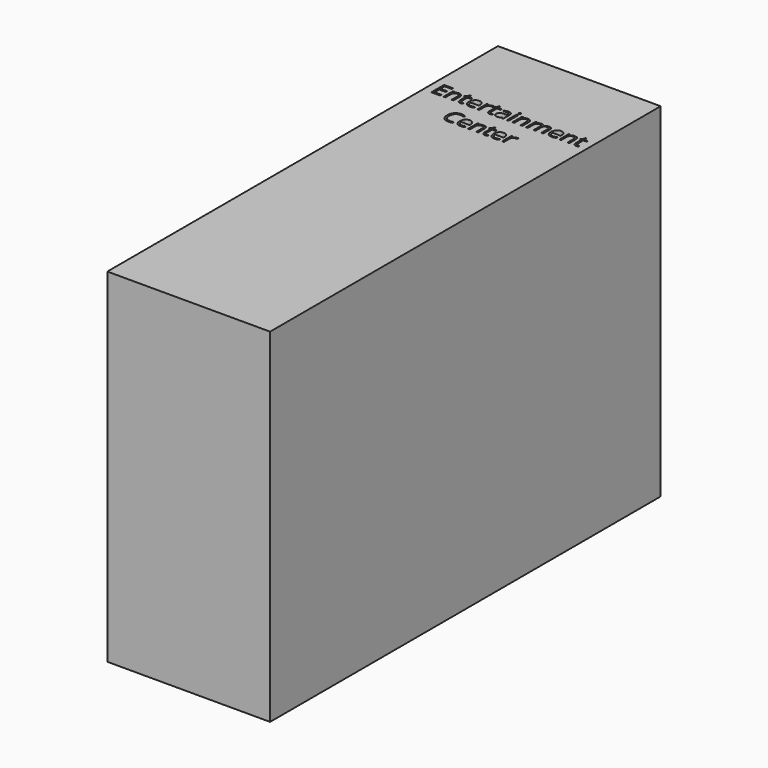
from build123d import *

# Parameters (mm, degrees)
F0_W     = 685.8
F0_H     = 2057.4
F0_W_2   = 7.6064578669
F0_H_2   = 50.1967595264
F1_DEPTH = 1447.8


with BuildPart() as f1:
    # F0 (on Top) → F1 (new body)
    with BuildSketch(Plane.XY):
        Rectangle(F0_W, F0_H)
        Polygon((-270.9672375193, 641.7474361589), (-270.9672375193, 634.785841772), (-308.2960394211, 634.785841772), (-308.2960394211, 701.7490517796), (-270.9672375193, 701.7490517796), (-270.9672375193, 694.8314253573), (-300.513709696, 694.8314253573), (-300.513709696, 673.2578107521), (-272.7552680776, 673.2578107521), (-272.7552680776, 666.3841522943), (-300.513709696, 666.3841522943), (-300.513709696, 641.7474361589), align=None, mode=Mode.SUBTRACT)
        with BuildLine():
            Line((-215.3184503889, 634.785841772), (-222.9249082558, 634.785841772))
            Line((-222.9249082558, 634.785841772), (-222.9249082558, 667.2635115853))
            add(Edge.make_bspline(
                [(-222.9249082558, 667.2635115853), (-222.9249082558, 673.3897146457), (-225.7168740047, 676.4161762055)],
                knots=[0, 0, 0, 1, 1, 1], degree=2))
            add(Edge.make_bspline(
                [(-225.7168740047, 676.4161762055), (-228.5088397535, 679.4426377653), (-234.4738269439, 679.4426377653)],
                knots=[0, 0, 0, 1, 1, 1], degree=2))
            add(Edge.make_bspline(
                [(-234.4738269439, 679.4426377653), (-242.3440925981, 679.4426377653), (-246.0080896439, 675.1850731981)],
                knots=[0, 0, 0, 1, 1, 1], degree=2))
            add(Edge.make_bspline(
                [(-246.0080896439, 675.1850731981), (-249.6720866896, 670.927508631), (-249.6720866896, 661.1226525367)],
                knots=[0, 0, 0, 1, 1, 1], degree=2))
            Line((-249.6720866896, 661.1226525367), (-249.6720866896, 634.785841772))
            Line((-249.6720866896, 634.785841772), (-257.2785445565, 634.785841772))
            Line((-257.2785445565, 634.785841772), (-257.2785445565, 684.9826012984))
            Line((-257.2785445565, 684.9826012984), (-251.0937175433, 684.9826012984))
            Line((-251.0937175433, 684.9826012984), (-249.862614536, 678.1089428406))
            Line((-249.862614536, 678.1089428406), (-249.4962148314, 678.1089428406))
            add(Edge.make_bspline(
                [(-249.4962148314, 678.1089428406), (-247.1512567221, 681.8169078509), (-242.9376601196, 683.8614182024)],
                knots=[0, 0, 0, 1, 1, 1], degree=2))
            add(Edge.make_bspline(
                [(-242.9376601196, 683.8614182024), (-238.724063517, 685.9059285539), (-233.5504996884, 685.9059285539)],
                knots=[0, 0, 0, 1, 1, 1], degree=2))
            add(Edge.make_bspline(
                [(-233.5504996884, 685.9059285539), (-224.4784430032, 685.9059285539), (-219.8984466961, 681.5311160813)],
                knots=[0, 0, 0, 1, 1, 1], degree=2))
            add(Edge.make_bspline(
                [(-219.8984466961, 681.5311160813), (-215.3184503889, 677.1563036087), (-215.3184503889, 667.5273193726)],
                knots=[0, 0, 0, 1, 1, 1], degree=2))
            Line((-215.3184503889, 667.5273193726), (-215.3184503889, 634.785841772))
        make_face(mode=Mode.SUBTRACT)
        with BuildLine():
            add(Edge.make_bspline(
                [(-189.4066632816, 642.5754994912), (-187.2522330187, 640.1499334469), (-183.5003000439, 640.1499334469)],
                knots=[0, 0, 0, 1, 1, 1], degree=2))
            add(Edge.make_bspline(
                [(-183.5003000439, 640.1499334469), (-181.4777736746, 640.1499334469), (-179.6018071872, 640.4430532106)],
                knots=[0, 0, 0, 1, 1, 1], degree=2))
            add(Edge.make_bspline(
                [(-179.6018071872, 640.4430532106), (-177.7258406998, 640.7361729743), (-176.6266415861, 641.0586047143)],
                knots=[0, 0, 0, 1, 1, 1], degree=2))
            Line((-176.6266415861, 641.0586047143), (-176.6266415861, 635.2401774057))
            add(Edge.make_bspline(
                [(-176.6266415861, 635.2401774057), (-177.8577445934, 634.6539378784), (-180.2613266554, 634.2582261974)],
                knots=[0, 0, 0, 1, 1, 1], degree=2))
            add(Edge.make_bspline(
                [(-180.2613266554, 634.2582261974), (-182.6649087174, 633.8625145165), (-184.5994991576, 633.8625145165)],
                knots=[0, 0, 0, 1, 1, 1], degree=2))
            add(Edge.make_bspline(
                [(-184.5994991576, 633.8625145165), (-199.1528954232, 633.8625145165), (-199.1528954232, 649.207334144)],
                knots=[0, 0, 0, 1, 1, 1], degree=2))
            Line((-199.1528954232, 649.207334144), (-199.1528954232, 679.0762380607))
            Line((-199.1528954232, 679.0762380607), (-206.348985621, 679.0762380607))
            Line((-206.348985621, 679.0762380607), (-206.348985621, 682.7402351064))
            Line((-206.348985621, 682.7402351064), (-199.1528954232, 685.9059285539))
            Line((-199.1528954232, 685.9059285539), (-195.9578899993, 696.6194559156))
            Line((-195.9578899993, 696.6194559156), (-191.5610935444, 696.6194559156))
            Line((-191.5610935444, 696.6194559156), (-191.5610935444, 684.9826012984))
            Line((-191.5610935444, 684.9826012984), (-176.9930412907, 684.9826012984))
            Line((-176.9930412907, 684.9826012984), (-176.9930412907, 679.0762380607))
            Line((-176.9930412907, 679.0762380607), (-191.5610935444, 679.0762380607))
            Line((-191.5610935444, 679.0762380607), (-191.5610935444, 649.529765884))
            add(Edge.make_bspline(
                [(-191.5610935444, 649.529765884), (-191.5610935444, 645.0010655355), (-189.4066632816, 642.5754994912)],
                knots=[0, 0, 0, 1, 1, 1], degree=2))
        make_face(mode=Mode.SUBTRACT)
        with BuildLine():
            add(Edge.make_bspline(
                [(-118.1785607127, 564.6129703523), (-125.7850185796, 568.1743754808), (-133.3914764466, 568.1743754808)],
                knots=[0, 0, 0, 1, 1, 1], degree=2))
            add(Edge.make_bspline(
                [(-133.3914764466, 568.1743754808), (-144.4274355483, 568.1743754808), (-150.817446396, 560.8243974071)],
                knots=[0, 0, 0, 1, 1, 1], degree=2))
            add(Edge.make_bspline(
                [(-150.817446396, 560.8243974071), (-157.2074572438, 553.4744193333), (-157.2074572438, 540.6943976379)],
                knots=[0, 0, 0, 1, 1, 1], degree=2))
            add(Edge.make_bspline(
                [(-157.2074572438, 540.6943976379), (-157.2074572438, 527.562632226), (-151.0446142128, 520.3885260105)],
                knots=[0, 0, 0, 1, 1, 1], degree=2))
            add(Edge.make_bspline(
                [(-151.0446142128, 520.3885260105), (-144.8817711819, 513.2144197949), (-133.4794123757, 513.2144197949)],
                knots=[0, 0, 0, 1, 1, 1], degree=2))
            add(Edge.make_bspline(
                [(-133.4794123757, 513.2144197949), (-126.4738500242, 513.2144197949), (-117.4897292681, 515.7352497624)],
                knots=[0, 0, 0, 1, 1, 1], degree=2))
            Line((-117.4897292681, 515.7352497624), (-117.4897292681, 508.9202152574))
            add(Edge.make_bspline(
                [(-117.4897292681, 508.9202152574), (-124.451323655, 506.2967933726), (-134.6665474185, 506.2967933726)],
                knots=[0, 0, 0, 1, 1, 1], degree=2))
            add(Edge.make_bspline(
                [(-134.6665474185, 506.2967933726), (-149.454439495, 506.2967933726), (-157.4932490133, 515.2809141287)],
                knots=[0, 0, 0, 1, 1, 1], degree=2))
            add(Edge.make_bspline(
                [(-157.4932490133, 515.2809141287), (-165.5320585316, 524.2650348848), (-165.5320585316, 540.7969895551)],
                knots=[0, 0, 0, 1, 1, 1], degree=2))
            add(Edge.make_bspline(
                [(-165.5320585316, 540.7969895551), (-165.5320585316, 551.1441172123), (-161.6628776513, 558.9264469374)],
                knots=[0, 0, 0, 1, 1, 1], degree=2))
            add(Edge.make_bspline(
                [(-161.6628776513, 558.9264469374), (-157.7936967711, 566.7087766625), (-150.4876866619, 570.9223732651)],
                knots=[0, 0, 0, 1, 1, 1], degree=2))
            add(Edge.make_bspline(
                [(-150.4876866619, 570.9223732651), (-143.1816765527, 575.1359698677), (-133.2888845293, 575.1359698677)],
                knots=[0, 0, 0, 1, 1, 1], degree=2))
            add(Edge.make_bspline(
                [(-133.2888845293, 575.1359698677), (-122.765885014, 575.1359698677), (-114.8809633716, 571.2961009637)],
                knots=[0, 0, 0, 1, 1, 1], degree=2))
            Line((-114.8809633716, 571.2961009637), (-118.1785607127, 564.6129703523))
        make_face(mode=Mode.SUBTRACT)
        with BuildLine():
            add(Edge.make_bspline(
                [(-136.7183857641, 634.624625902), (-140.3091028689, 633.8625145165), (-145.3947307683, 633.8625145165)],
                knots=[0, 0, 0, 1, 1, 1], degree=2))
            add(Edge.make_bspline(
                [(-145.3947307683, 633.8625145165), (-156.5186257992, 633.8625145165), (-162.9599326055, 640.6482370452)],
                knots=[0, 0, 0, 1, 1, 1], degree=2))
            add(Edge.make_bspline(
                [(-162.9599326055, 640.6482370452), (-169.4012394119, 647.4339595738), (-169.4012394119, 659.466525872)],
                knots=[0, 0, 0, 1, 1, 1], degree=2))
            add(Edge.make_bspline(
                [(-169.4012394119, 659.466525872), (-169.4012394119, 671.6163400756), (-163.4215962333, 678.7611343148)],
                knots=[0, 0, 0, 1, 1, 1], degree=2))
            add(Edge.make_bspline(
                [(-163.4215962333, 678.7611343148), (-157.4419530547, 685.9059285539), (-147.3586331849, 685.9059285539)],
                knots=[0, 0, 0, 1, 1, 1], degree=2))
            add(Edge.make_bspline(
                [(-147.3586331849, 685.9059285539), (-137.9348327833, 685.9059285539), (-132.4388372147, 679.6991175585)],
                knots=[0, 0, 0, 1, 1, 1], degree=2))
            add(Edge.make_bspline(
                [(-132.4388372147, 679.6991175585), (-126.9428416461, 673.492306563), (-126.9428416461, 663.3210507641)],
                knots=[0, 0, 0, 1, 1, 1], degree=2))
            Line((-126.9428416461, 663.3210507641), (-126.9428416461, 658.5138866401))
            Line((-126.9428416461, 658.5138866401), (-161.5163177695, 658.5138866401))
            add(Edge.make_bspline(
                [(-161.5163177695, 658.5138866401), (-161.2818219586, 649.6763257658), (-157.0462413737, 645.0963294587)],
                knots=[0, 0, 0, 1, 1, 1], degree=2))
            add(Edge.make_bspline(
                [(-157.0462413737, 645.0963294587), (-152.8106607889, 640.5163331515), (-145.1162669929, 640.5163331515)],
                knots=[0, 0, 0, 1, 1, 1], degree=2))
            add(Edge.make_bspline(
                [(-145.1162669929, 640.5163331515), (-137.0115055277, 640.5163331515), (-129.097271909, 643.9018664218)],
                knots=[0, 0, 0, 1, 1, 1], degree=2))
            Line((-129.097271909, 643.9018664218), (-129.097271909, 637.1161438931))
            add(Edge.make_bspline(
                [(-129.097271909, 637.1161438931), (-133.1276686593, 635.3867372875), (-136.7183857641, 634.624625902)],
                knots=[0, 0, 0, 1, 1, 1], degree=2))
        make_face(mode=Mode.SUBTRACT)
        with BuildLine():
            add(Edge.make_bspline(
                [(-99.7266715905, 683.2458666987), (-95.7842107693, 685.9059285539), (-91.0649825744, 685.9059285539)],
                knots=[0, 0, 0, 1, 1, 1], degree=2))
            add(Edge.make_bspline(
                [(-91.0649825744, 685.9059285539), (-87.7234172687, 685.9059285539), (-85.0706834076, 685.349001003)],
                knots=[0, 0, 0, 1, 1, 1], degree=2))
            Line((-85.0706834076, 685.349001003), (-86.1259145567, 678.299470687))
            add(Edge.make_bspline(
                [(-86.1259145567, 678.299470687), (-89.2329840515, 678.9883021316), (-91.6219101253, 678.9883021316)],
                knots=[0, 0, 0, 1, 1, 1], degree=2))
            add(Edge.make_bspline(
                [(-91.6219101253, 678.9883021316), (-97.7188012094, 678.9883021316), (-102.0423177234, 674.0419061199)],
                knots=[0, 0, 0, 1, 1, 1], degree=2))
            add(Edge.make_bspline(
                [(-102.0423177234, 674.0419061199), (-106.3658342373, 669.0955101081), (-106.3658342373, 661.7235480522)],
                knots=[0, 0, 0, 1, 1, 1], degree=2))
            Line((-106.3658342373, 661.7235480522), (-106.3658342373, 634.785841772))
            Line((-106.3658342373, 634.785841772), (-113.9722921042, 634.785841772))
            Line((-113.9722921042, 634.785841772), (-113.9722921042, 684.9826012984))
            Line((-113.9722921042, 684.9826012984), (-107.699529162, 684.9826012984))
            Line((-107.699529162, 684.9826012984), (-106.820169871, 675.6907047904))
            Line((-106.820169871, 675.6907047904), (-106.4537701664, 675.6907047904))
            add(Edge.make_bspline(
                [(-106.4537701664, 675.6907047904), (-103.6691324117, 680.5858048435), (-99.7266715905, 683.2458666987)],
                knots=[0, 0, 0, 1, 1, 1], degree=2))
        make_face(mode=Mode.SUBTRACT)
        with BuildLine():
            add(Edge.make_bspline(
                [(-74.1373162231, 507.0589047581), (-77.7280333279, 506.2967933726), (-82.8136612274, 506.2967933726)],
                knots=[0, 0, 0, 1, 1, 1], degree=2))
            add(Edge.make_bspline(
                [(-82.8136612274, 506.2967933726), (-93.9375562582, 506.2967933726), (-100.3788630646, 513.0825159013)],
                knots=[0, 0, 0, 1, 1, 1], degree=2))
            add(Edge.make_bspline(
                [(-100.3788630646, 513.0825159013), (-106.820169871, 519.86823843), (-106.820169871, 531.9008047281)],
                knots=[0, 0, 0, 1, 1, 1], degree=2))
            add(Edge.make_bspline(
                [(-106.820169871, 531.9008047281), (-106.820169871, 544.0506189317), (-100.8405266924, 551.1954131709)],
                knots=[0, 0, 0, 1, 1, 1], degree=2))
            add(Edge.make_bspline(
                [(-100.8405266924, 551.1954131709), (-94.8608835137, 558.3402074101), (-84.7775636439, 558.3402074101)],
                knots=[0, 0, 0, 1, 1, 1], degree=2))
            add(Edge.make_bspline(
                [(-84.7775636439, 558.3402074101), (-75.3537632423, 558.3402074101), (-69.8577676737, 552.1333964146)],
                knots=[0, 0, 0, 1, 1, 1], degree=2))
            add(Edge.make_bspline(
                [(-69.8577676737, 552.1333964146), (-64.3617721052, 545.9265854192), (-64.3617721052, 535.7553296202)],
                knots=[0, 0, 0, 1, 1, 1], degree=2))
            Line((-64.3617721052, 535.7553296202), (-64.3617721052, 530.9481654962))
            Line((-64.3617721052, 530.9481654962), (-98.9352482286, 530.9481654962))
            add(Edge.make_bspline(
                [(-98.9352482286, 530.9481654962), (-98.7007524177, 522.110604622), (-94.4651718328, 517.5306083148)],
                knots=[0, 0, 0, 1, 1, 1], degree=2))
            add(Edge.make_bspline(
                [(-94.4651718328, 517.5306083148), (-90.229591248, 512.9506120077), (-82.5351974519, 512.9506120077)],
                knots=[0, 0, 0, 1, 1, 1], degree=2))
            add(Edge.make_bspline(
                [(-82.5351974519, 512.9506120077), (-74.4304359868, 512.9506120077), (-66.516202368, 516.3361452779)],
                knots=[0, 0, 0, 1, 1, 1], degree=2))
            Line((-66.516202368, 516.3361452779), (-66.516202368, 509.5504227492))
            add(Edge.make_bspline(
                [(-66.516202368, 509.5504227492), (-70.5465991183, 507.8210161436), (-74.1373162231, 507.0589047581)],
                knots=[0, 0, 0, 1, 1, 1], degree=2))
        make_face(mode=Mode.SUBTRACT)
        with BuildLine():
            Line((-9.4311283957, 507.2201206281), (-17.0375862626, 507.2201206281))
            Line((-17.0375862626, 507.2201206281), (-17.0375862626, 539.6977904414))
            add(Edge.make_bspline(
                [(-17.0375862626, 539.6977904414), (-17.0375862626, 545.8239935019), (-19.8295520114, 548.8504550616)],
                knots=[0, 0, 0, 1, 1, 1], degree=2))
            add(Edge.make_bspline(
                [(-19.8295520114, 548.8504550616), (-22.6215177603, 551.8769166214), (-28.5865049507, 551.8769166214)],
                knots=[0, 0, 0, 1, 1, 1], degree=2))
            add(Edge.make_bspline(
                [(-28.5865049507, 551.8769166214), (-36.4567706049, 551.8769166214), (-40.1207676507, 547.6193520543)],
                knots=[0, 0, 0, 1, 1, 1], degree=2))
            add(Edge.make_bspline(
                [(-40.1207676507, 547.6193520543), (-43.7847646964, 543.3617874871), (-43.7847646964, 533.5569313928)],
                knots=[0, 0, 0, 1, 1, 1], degree=2))
            Line((-43.7847646964, 533.5569313928), (-43.7847646964, 507.2201206281))
            Line((-43.7847646964, 507.2201206281), (-51.3912225633, 507.2201206281))
            Line((-51.3912225633, 507.2201206281), (-51.3912225633, 557.4168801545))
            Line((-51.3912225633, 557.4168801545), (-45.2063955501, 557.4168801545))
            Line((-45.2063955501, 557.4168801545), (-43.9752925428, 550.5432216968))
            Line((-43.9752925428, 550.5432216968), (-43.6088928382, 550.5432216968))
            add(Edge.make_bspline(
                [(-43.6088928382, 550.5432216968), (-41.2639347289, 554.251186707), (-37.0503381263, 556.2956970585)],
                knots=[0, 0, 0, 1, 1, 1], degree=2))
            add(Edge.make_bspline(
                [(-37.0503381263, 556.2956970585), (-32.8367415238, 558.3402074101), (-27.6631776952, 558.3402074101)],
                knots=[0, 0, 0, 1, 1, 1], degree=2))
            add(Edge.make_bspline(
                [(-27.6631776952, 558.3402074101), (-18.59112101, 558.3402074101), (-14.0111247028, 553.9653949375)],
                knots=[0, 0, 0, 1, 1, 1], degree=2))
            add(Edge.make_bspline(
                [(-14.0111247028, 553.9653949375), (-9.4311283957, 549.5905824649), (-9.4311283957, 539.9615982287)],
                knots=[0, 0, 0, 1, 1, 1], degree=2))
            Line((-9.4311283957, 539.9615982287), (-9.4311283957, 507.2201206281))
        make_face(mode=Mode.SUBTRACT)
        with BuildLine():
            add(Edge.make_bspline(
                [(-65.3730352898, 642.5754994912), (-63.2186050269, 640.1499334469), (-59.4666720521, 640.1499334469)],
                knots=[0, 0, 0, 1, 1, 1], degree=2))
            add(Edge.make_bspline(
                [(-59.4666720521, 640.1499334469), (-57.4441456828, 640.1499334469), (-55.5681791954, 640.4430532106)],
                knots=[0, 0, 0, 1, 1, 1], degree=2))
            add(Edge.make_bspline(
                [(-55.5681791954, 640.4430532106), (-53.692212708, 640.7361729743), (-52.5930135943, 641.0586047143)],
                knots=[0, 0, 0, 1, 1, 1], degree=2))
            Line((-52.5930135943, 641.0586047143), (-52.5930135943, 635.2401774057))
            add(Edge.make_bspline(
                [(-52.5930135943, 635.2401774057), (-53.8241166017, 634.6539378784), (-56.2276986637, 634.2582261974)],
                knots=[0, 0, 0, 1, 1, 1], degree=2))
            add(Edge.make_bspline(
                [(-56.2276986637, 634.2582261974), (-58.6312807256, 633.8625145165), (-60.5658711658, 633.8625145165)],
                knots=[0, 0, 0, 1, 1, 1], degree=2))
            add(Edge.make_bspline(
                [(-60.5658711658, 633.8625145165), (-75.1192674314, 633.8625145165), (-75.1192674314, 649.207334144)],
                knots=[0, 0, 0, 1, 1, 1], degree=2))
            Line((-75.1192674314, 649.207334144), (-75.1192674314, 679.0762380607))
            Line((-75.1192674314, 679.0762380607), (-82.3153576292, 679.0762380607))
            Line((-82.3153576292, 679.0762380607), (-82.3153576292, 682.7402351064))
            Line((-82.3153576292, 682.7402351064), (-75.1192674314, 685.9059285539))
            Line((-75.1192674314, 685.9059285539), (-71.9242620075, 696.6194559156))
            Line((-71.9242620075, 696.6194559156), (-67.5274655527, 696.6194559156))
            Line((-67.5274655527, 696.6194559156), (-67.5274655527, 684.9826012984))
            Line((-67.5274655527, 684.9826012984), (-52.9594132989, 684.9826012984))
            Line((-52.9594132989, 684.9826012984), (-52.9594132989, 679.0762380607))
            Line((-52.9594132989, 679.0762380607), (-67.5274655527, 679.0762380607))
            Line((-67.5274655527, 679.0762380607), (-67.5274655527, 649.529765884))
            add(Edge.make_bspline(
                [(-67.5274655527, 649.529765884), (-67.5274655527, 645.0010655355), (-65.3730352898, 642.5754994912)],
                knots=[0, 0, 0, 1, 1, 1], degree=2))
        make_face(mode=Mode.SUBTRACT)
        with BuildLine():
            Line((-6.0602511136, 634.785841772), (-11.702806564, 634.785841772))
            Line((-11.702806564, 634.785841772), (-13.2123733469, 641.9379640053))
            Line((-13.2123733469, 641.9379640053), (-13.5787730514, 641.9379640053))
            add(Edge.make_bspline(
                [(-13.5787730514, 641.9379640053), (-17.3307060263, 637.2187358104), (-21.0606550188, 635.5406251634)],
                knots=[0, 0, 0, 1, 1, 1], degree=2))
            add(Edge.make_bspline(
                [(-21.0606550188, 635.5406251634), (-24.7906040114, 633.8625145165), (-30.3891914972, 633.8625145165)],
                knots=[0, 0, 0, 1, 1, 1], degree=2))
            add(Edge.make_bspline(
                [(-30.3891914972, 633.8625145165), (-37.8490894823, 633.8625145165), (-42.0846700672, 637.7170394086)],
                knots=[0, 0, 0, 1, 1, 1], degree=2))
            add(Edge.make_bspline(
                [(-42.0846700672, 637.7170394086), (-46.320250652, 641.5715643007), (-46.320250652, 648.6650625812)],
                knots=[0, 0, 0, 1, 1, 1], degree=2))
            add(Edge.make_bspline(
                [(-46.320250652, 648.6650625812), (-46.320250652, 663.8633223269), (-22.0059662566, 664.596121736)],
                knots=[0, 0, 0, 1, 1, 1], degree=2))
            Line((-22.0059662566, 664.596121736), (-13.4908371223, 664.8745855115))
            Line((-13.4908371223, 664.8745855115), (-13.4908371223, 667.9963109944))
            add(Edge.make_bspline(
                [(-13.4908371223, 667.9963109944), (-13.4908371223, 673.9026742321), (-16.026323078, 676.7166239633)],
                knots=[0, 0, 0, 1, 1, 1], degree=2))
            add(Edge.make_bspline(
                [(-16.026323078, 676.7166239633), (-18.5618090336, 679.5305736944), (-24.1603965195, 679.5305736944)],
                knots=[0, 0, 0, 1, 1, 1], degree=2))
            add(Edge.make_bspline(
                [(-24.1603965195, 679.5305736944), (-30.4331594618, 679.5305736944), (-38.3473930805, 675.6907047904)],
                knots=[0, 0, 0, 1, 1, 1], degree=2))
            Line((-38.3473930805, 675.6907047904), (-40.6923511898, 681.5091320991))
            add(Edge.make_bspline(
                [(-40.6923511898, 681.5091320991), (-36.9843861795, 683.5170024801), (-32.5656057424, 684.6601695584)],
                knots=[0, 0, 0, 1, 1, 1], degree=2))
            add(Edge.make_bspline(
                [(-32.5656057424, 684.6601695584), (-28.1468253052, 685.8033366366), (-23.6914048976, 685.8033366366)],
                knots=[0, 0, 0, 1, 1, 1], degree=2))
            add(Edge.make_bspline(
                [(-23.6914048976, 685.8033366366), (-14.7219401297, 685.8033366366), (-10.3910956217, 681.824235845)],
                knots=[0, 0, 0, 1, 1, 1], degree=2))
            add(Edge.make_bspline(
                [(-10.3910956217, 681.824235845), (-6.0602511136, 677.8451350533), (-6.0602511136, 669.0515421436)],
                knots=[0, 0, 0, 1, 1, 1], degree=2))
            Line((-6.0602511136, 669.0515421436), (-6.0602511136, 634.785841772))
        make_face(mode=Mode.SUBTRACT)
        with BuildLine():
            add(Edge.make_bspline(
                [(16.4806587117, 515.0097783474), (18.6350889745, 512.5842123031), (22.3870219494, 512.5842123031)],
                knots=[0, 0, 0, 1, 1, 1], degree=2))
            add(Edge.make_bspline(
                [(22.3870219494, 512.5842123031), (24.4095483186, 512.5842123031), (26.285514806, 512.8773320667)],
                knots=[0, 0, 0, 1, 1, 1], degree=2))
            add(Edge.make_bspline(
                [(26.285514806, 512.8773320667), (28.1614812934, 513.1704518304), (29.2606804071, 513.4928835704)],
                knots=[0, 0, 0, 1, 1, 1], degree=2))
            Line((29.2606804071, 513.4928835704), (29.2606804071, 507.6744562618))
            add(Edge.make_bspline(
                [(29.2606804071, 507.6744562618), (28.0295773998, 507.0882167345), (25.6259953378, 506.6925050536)],
                knots=[0, 0, 0, 1, 1, 1], degree=2))
            add(Edge.make_bspline(
                [(25.6259953378, 506.6925050536), (23.2224132758, 506.2967933726), (21.2878228356, 506.2967933726)],
                knots=[0, 0, 0, 1, 1, 1], degree=2))
            add(Edge.make_bspline(
                [(21.2878228356, 506.2967933726), (6.73442657, 506.2967933726), (6.73442657, 521.6416130001)],
                knots=[0, 0, 0, 1, 1, 1], degree=2))
            Line((6.73442657, 521.6416130001), (6.73442657, 551.5105169168))
            Line((6.73442657, 551.5105169168), (-0.4616636278, 551.5105169168))
            Line((-0.4616636278, 551.5105169168), (-0.4616636278, 555.1745139626))
            Line((-0.4616636278, 555.1745139626), (6.73442657, 558.3402074101))
            Line((6.73442657, 558.3402074101), (9.9294319939, 569.0537347718))
            Line((9.9294319939, 569.0537347718), (14.3262284488, 569.0537347718))
            Line((14.3262284488, 569.0537347718), (14.3262284488, 557.4168801545))
            Line((14.3262284488, 557.4168801545), (28.8942807026, 557.4168801545))
            Line((28.8942807026, 557.4168801545), (28.8942807026, 551.5105169168))
            Line((28.8942807026, 551.5105169168), (14.3262284488, 551.5105169168))
            Line((14.3262284488, 551.5105169168), (14.3262284488, 521.9640447401))
            add(Edge.make_bspline(
                [(14.3262284488, 521.9640447401), (14.3262284488, 517.4353443916), (16.4806587117, 515.0097783474)],
                knots=[0, 0, 0, 1, 1, 1], degree=2))
        make_face(mode=Mode.SUBTRACT)
        with BuildLine():
            add(Edge.make_bspline(
                [(69.1689362291, 507.0589047581), (65.5782191243, 506.2967933726), (60.4925912249, 506.2967933726)],
                knots=[0, 0, 0, 1, 1, 1], degree=2))
            add(Edge.make_bspline(
                [(60.4925912249, 506.2967933726), (49.3686961941, 506.2967933726), (42.9273893877, 513.0825159013)],
                knots=[0, 0, 0, 1, 1, 1], degree=2))
            add(Edge.make_bspline(
                [(42.9273893877, 513.0825159013), (36.4860825813, 519.86823843), (36.4860825813, 531.9008047281)],
                knots=[0, 0, 0, 1, 1, 1], degree=2))
            add(Edge.make_bspline(
                [(36.4860825813, 531.9008047281), (36.4860825813, 544.0506189317), (42.4657257599, 551.1954131709)],
                knots=[0, 0, 0, 1, 1, 1], degree=2))
            add(Edge.make_bspline(
                [(42.4657257599, 551.1954131709), (48.4453689385, 558.3402074101), (58.5286888084, 558.3402074101)],
                knots=[0, 0, 0, 1, 1, 1], degree=2))
            add(Edge.make_bspline(
                [(58.5286888084, 558.3402074101), (67.95248921, 558.3402074101), (73.4484847785, 552.1333964146)],
                knots=[0, 0, 0, 1, 1, 1], degree=2))
            add(Edge.make_bspline(
                [(73.4484847785, 552.1333964146), (78.9444803471, 545.9265854192), (78.9444803471, 535.7553296202)],
                knots=[0, 0, 0, 1, 1, 1], degree=2))
            Line((78.9444803471, 535.7553296202), (78.9444803471, 530.9481654962))
            Line((78.9444803471, 530.9481654962), (44.3710042237, 530.9481654962))
            add(Edge.make_bspline(
                [(44.3710042237, 530.9481654962), (44.6055000346, 522.110604622), (48.8410806195, 517.5306083148)],
                knots=[0, 0, 0, 1, 1, 1], degree=2))
            add(Edge.make_bspline(
                [(48.8410806195, 517.5306083148), (53.0766612043, 512.9506120077), (60.7710550003, 512.9506120077)],
                knots=[0, 0, 0, 1, 1, 1], degree=2))
            add(Edge.make_bspline(
                [(60.7710550003, 512.9506120077), (68.8758164655, 512.9506120077), (76.7900500842, 516.3361452779)],
                knots=[0, 0, 0, 1, 1, 1], degree=2))
            Line((76.7900500842, 516.3361452779), (76.7900500842, 509.5504227492))
            add(Edge.make_bspline(
                [(76.7900500842, 509.5504227492), (72.7596533339, 507.8210161436), (69.1689362291, 507.0589047581)],
                knots=[0, 0, 0, 1, 1, 1], degree=2))
        make_face(mode=Mode.SUBTRACT)
        with Locations((13.3955731992, 659.8842215352)):
            Rectangle(F0_W_2, F0_H_2, mode=Mode.SUBTRACT)
        with BuildLine():
            add(Edge.make_bspline(
                [(10.2298797517, 694.7581454164), (8.9474807857, 696.0185604001), (8.9474807857, 698.5833583321)],
                knots=[0, 0, 0, 1, 1, 1], degree=2))
            add(Edge.make_bspline(
                [(8.9474807857, 698.5833583321), (8.9474807857, 701.1921242287), (10.2298797517, 702.4085712479)],
                knots=[0, 0, 0, 1, 1, 1], degree=2))
            add(Edge.make_bspline(
                [(10.2298797517, 702.4085712479), (11.5122787177, 703.625018267), (13.4468691578, 703.625018267)],
                knots=[0, 0, 0, 1, 1, 1], degree=2))
            add(Edge.make_bspline(
                [(13.4468691578, 703.625018267), (15.2788676807, 703.625018267), (16.6052346112, 702.3865872656)],
                knots=[0, 0, 0, 1, 1, 1], degree=2))
            add(Edge.make_bspline(
                [(16.6052346112, 702.3865872656), (17.9316015418, 701.1481562641), (17.9316015418, 698.5833583321)],
                knots=[0, 0, 0, 1, 1, 1], degree=2))
            add(Edge.make_bspline(
                [(17.9316015418, 698.5833583321), (17.9316015418, 696.0185604001), (16.6052346112, 694.7581454164)],
                knots=[0, 0, 0, 1, 1, 1], degree=2))
            add(Edge.make_bspline(
                [(16.6052346112, 694.7581454164), (15.2788676807, 693.4977304327), (13.4468691578, 693.4977304327)],
                knots=[0, 0, 0, 1, 1, 1], degree=2))
            add(Edge.make_bspline(
                [(13.4468691578, 693.4977304327), (11.5122787177, 693.4977304327), (10.2298797517, 694.7581454164)],
                knots=[0, 0, 0, 1, 1, 1], degree=2))
        make_face(mode=Mode.SUBTRACT)
        with BuildLine():
            Line((75.2804833014, 634.785841772), (67.6740254345, 634.785841772))
            Line((67.6740254345, 634.785841772), (67.6740254345, 667.2635115853))
            add(Edge.make_bspline(
                [(67.6740254345, 667.2635115853), (67.6740254345, 673.3897146457), (64.8820596856, 676.4161762055)],
                knots=[0, 0, 0, 1, 1, 1], degree=2))
            add(Edge.make_bspline(
                [(64.8820596856, 676.4161762055), (62.0900939368, 679.4426377653), (56.1251067464, 679.4426377653)],
                knots=[0, 0, 0, 1, 1, 1], degree=2))
            add(Edge.make_bspline(
                [(56.1251067464, 679.4426377653), (48.2548410922, 679.4426377653), (44.5908440464, 675.1850731981)],
                knots=[0, 0, 0, 1, 1, 1], degree=2))
            add(Edge.make_bspline(
                [(44.5908440464, 675.1850731981), (40.9268470007, 670.927508631), (40.9268470007, 661.1226525367)],
                knots=[0, 0, 0, 1, 1, 1], degree=2))
            Line((40.9268470007, 661.1226525367), (40.9268470007, 634.785841772))
            Line((40.9268470007, 634.785841772), (33.3203891338, 634.785841772))
            Line((33.3203891338, 634.785841772), (33.3203891338, 684.9826012984))
            Line((33.3203891338, 684.9826012984), (39.505216147, 684.9826012984))
            Line((39.505216147, 684.9826012984), (40.7363191543, 678.1089428406))
            Line((40.7363191543, 678.1089428406), (41.1027188589, 678.1089428406))
            add(Edge.make_bspline(
                [(41.1027188589, 678.1089428406), (43.4476769682, 681.8169078509), (47.6612735708, 683.8614182024)],
                knots=[0, 0, 0, 1, 1, 1], degree=2))
            add(Edge.make_bspline(
                [(47.6612735708, 683.8614182024), (51.8748701733, 685.9059285539), (57.0484340019, 685.9059285539)],
                knots=[0, 0, 0, 1, 1, 1], degree=2))
            add(Edge.make_bspline(
                [(57.0484340019, 685.9059285539), (66.1204906871, 685.9059285539), (70.7004869943, 681.5311160813)],
                knots=[0, 0, 0, 1, 1, 1], degree=2))
            add(Edge.make_bspline(
                [(70.7004869943, 681.5311160813), (75.2804833014, 677.1563036087), (75.2804833014, 667.5273193726)],
                knots=[0, 0, 0, 1, 1, 1], degree=2))
            Line((75.2804833014, 667.5273193726), (75.2804833014, 634.785841772))
        make_face(mode=Mode.SUBTRACT)
        with BuildLine():
            add(Edge.make_bspline(
                [(106.1606504028, 555.6801455549), (110.1031112239, 558.3402074101), (114.8223394188, 558.3402074101)],
                knots=[0, 0, 0, 1, 1, 1], degree=2))
            add(Edge.make_bspline(
                [(114.8223394188, 558.3402074101), (118.1639047245, 558.3402074101), (120.8166385856, 557.7832798591)],
                knots=[0, 0, 0, 1, 1, 1], degree=2))
            Line((120.8166385856, 557.7832798591), (119.7614074365, 550.7337495431))
            add(Edge.make_bspline(
                [(119.7614074365, 550.7337495431), (116.6543379417, 551.4225809877), (114.2654118679, 551.4225809877)],
                knots=[0, 0, 0, 1, 1, 1], degree=2))
            add(Edge.make_bspline(
                [(114.2654118679, 551.4225809877), (108.1685207838, 551.4225809877), (103.8450042699, 546.476184976)],
                knots=[0, 0, 0, 1, 1, 1], degree=2))
            add(Edge.make_bspline(
                [(103.8450042699, 546.476184976), (99.5214877559, 541.5297889643), (99.5214877559, 534.1578269083)],
                knots=[0, 0, 0, 1, 1, 1], degree=2))
            Line((99.5214877559, 534.1578269083), (99.5214877559, 507.2201206281))
            Line((99.5214877559, 507.2201206281), (91.915029889, 507.2201206281))
            Line((91.915029889, 507.2201206281), (91.915029889, 557.4168801545))
            Line((91.915029889, 557.4168801545), (98.1877928313, 557.4168801545))
            Line((98.1877928313, 557.4168801545), (99.0671521222, 548.1249836466))
            Line((99.0671521222, 548.1249836466), (99.4335518268, 548.1249836466))
            add(Edge.make_bspline(
                [(99.4335518268, 548.1249836466), (102.2181895816, 553.0200836997), (106.1606504028, 555.6801455549)],
                knots=[0, 0, 0, 1, 1, 1], degree=2))
        make_face(mode=Mode.SUBTRACT)
        with BuildLine():
            Line((162.4689570014, 634.785841772), (154.8771551227, 634.785841772))
            Line((154.8771551227, 634.785841772), (154.8771551227, 667.4393834435))
            add(Edge.make_bspline(
                [(154.8771551227, 667.4393834435), (154.8771551227, 673.4483385985), (152.3123571907, 676.4454881819)],
                knots=[0, 0, 0, 1, 1, 1], degree=2))
            add(Edge.make_bspline(
                [(152.3123571907, 676.4454881819), (149.7475592587, 679.4426377653), (144.3394996192, 679.4426377653)],
                knots=[0, 0, 0, 1, 1, 1], degree=2))
            add(Edge.make_bspline(
                [(144.3394996192, 679.4426377653), (137.2460013387, 679.4426377653), (133.8531400743, 675.3682730504)],
                knots=[0, 0, 0, 1, 1, 1], degree=2))
            add(Edge.make_bspline(
                [(133.8531400743, 675.3682730504), (130.46027881, 671.2939083356), (130.46027881, 662.8227471659)],
                knots=[0, 0, 0, 1, 1, 1], degree=2))
            Line((130.46027881, 662.8227471659), (130.46027881, 634.785841772))
            Line((130.46027881, 634.785841772), (122.8538209431, 634.785841772))
            Line((122.8538209431, 634.785841772), (122.8538209431, 667.4393834435))
            add(Edge.make_bspline(
                [(122.8538209431, 667.4393834435), (122.8538209431, 673.4483385985), (120.2890230111, 676.4454881819)],
                knots=[0, 0, 0, 1, 1, 1], degree=2))
            add(Edge.make_bspline(
                [(120.2890230111, 676.4454881819), (117.7242250791, 679.4426377653), (112.272197475, 679.4426377653)],
                knots=[0, 0, 0, 1, 1, 1], degree=2))
            add(Edge.make_bspline(
                [(112.272197475, 679.4426377653), (105.1347312299, 679.4426377653), (101.8151499065, 675.1630892159)],
                knots=[0, 0, 0, 1, 1, 1], degree=2))
            add(Edge.make_bspline(
                [(101.8151499065, 675.1630892159), (98.4955685831, 670.8835406665), (98.4955685831, 661.1226525367)],
                knots=[0, 0, 0, 1, 1, 1], degree=2))
            Line((98.4955685831, 661.1226525367), (98.4955685831, 634.785841772))
            Line((98.4955685831, 634.785841772), (90.8891107162, 634.785841772))
            Line((90.8891107162, 634.785841772), (90.8891107162, 684.9826012984))
            Line((90.8891107162, 684.9826012984), (97.0739377294, 684.9826012984))
            Line((97.0739377294, 684.9826012984), (98.3050407367, 678.1089428406))
            Line((98.3050407367, 678.1089428406), (98.6714404413, 678.1089428406))
            add(Edge.make_bspline(
                [(98.6714404413, 678.1089428406), (100.8258707042, 681.7729398863), (104.7463475431, 683.8394342201)],
                knots=[0, 0, 0, 1, 1, 1], degree=2))
            add(Edge.make_bspline(
                [(104.7463475431, 683.8394342201), (108.666824382, 685.9059285539), (113.5179564706, 685.9059285539)],
                knots=[0, 0, 0, 1, 1, 1], degree=2))
            add(Edge.make_bspline(
                [(113.5179564706, 685.9059285539), (125.2867149814, 685.9059285539), (128.9067440626, 677.3761434315)],
                knots=[0, 0, 0, 1, 1, 1], degree=2))
            Line((128.9067440626, 677.3761434315), (129.2731437672, 677.3761434315))
            add(Edge.make_bspline(
                [(129.2731437672, 677.3761434315), (131.5155099591, 681.3186042527), (135.7730745263, 683.6122664033)],
                knots=[0, 0, 0, 1, 1, 1], degree=2))
            add(Edge.make_bspline(
                [(135.7730745263, 683.6122664033), (140.0306390934, 685.9059285539), (145.4826666974, 685.9059285539)],
                knots=[0, 0, 0, 1, 1, 1], degree=2))
            add(Edge.make_bspline(
                [(145.4826666974, 685.9059285539), (153.9977958317, 685.9059285539), (158.2333764166, 681.5311160813)],
                knots=[0, 0, 0, 1, 1, 1], degree=2))
            add(Edge.make_bspline(
                [(158.2333764166, 681.5311160813), (162.4689570014, 677.1563036087), (162.4689570014, 667.5273193726)],
                knots=[0, 0, 0, 1, 1, 1], degree=2))
            Line((162.4689570014, 667.5273193726), (162.4689570014, 634.785841772))
        make_face(mode=Mode.SUBTRACT)
        with BuildLine():
            add(Edge.make_bspline(
                [(208.0197682738, 634.624625902), (204.429051169, 633.8625145165), (199.3434232696, 633.8625145165)],
                knots=[0, 0, 0, 1, 1, 1], degree=2))
            add(Edge.make_bspline(
                [(199.3434232696, 633.8625145165), (188.2195282387, 633.8625145165), (181.7782214324, 640.6482370452)],
                knots=[0, 0, 0, 1, 1, 1], degree=2))
            add(Edge.make_bspline(
                [(181.7782214324, 640.6482370452), (175.336914626, 647.4339595738), (175.336914626, 659.466525872)],
                knots=[0, 0, 0, 1, 1, 1], degree=2))
            add(Edge.make_bspline(
                [(175.336914626, 659.466525872), (175.336914626, 671.6163400756), (181.3165578046, 678.7611343148)],
                knots=[0, 0, 0, 1, 1, 1], degree=2))
            add(Edge.make_bspline(
                [(181.3165578046, 678.7611343148), (187.2962009832, 685.9059285539), (197.379520853, 685.9059285539)],
                knots=[0, 0, 0, 1, 1, 1], degree=2))
            add(Edge.make_bspline(
                [(197.379520853, 685.9059285539), (206.8033212546, 685.9059285539), (212.2993168232, 679.6991175585)],
                knots=[0, 0, 0, 1, 1, 1], degree=2))
            add(Edge.make_bspline(
                [(212.2993168232, 679.6991175585), (217.7953123918, 673.492306563), (217.7953123918, 663.3210507641)],
                knots=[0, 0, 0, 1, 1, 1], degree=2))
            Line((217.7953123918, 663.3210507641), (217.7953123918, 658.5138866401))
            Line((217.7953123918, 658.5138866401), (183.2218362684, 658.5138866401))
            add(Edge.make_bspline(
                [(183.2218362684, 658.5138866401), (183.4563320793, 649.6763257658), (187.6919126642, 645.0963294587)],
                knots=[0, 0, 0, 1, 1, 1], degree=2))
            add(Edge.make_bspline(
                [(187.6919126642, 645.0963294587), (191.927493249, 640.5163331515), (199.621887045, 640.5163331515)],
                knots=[0, 0, 0, 1, 1, 1], degree=2))
            add(Edge.make_bspline(
                [(199.621887045, 640.5163331515), (207.7266485102, 640.5163331515), (215.6408821289, 643.9018664218)],
                knots=[0, 0, 0, 1, 1, 1], degree=2))
            Line((215.6408821289, 643.9018664218), (215.6408821289, 637.1161438931))
            add(Edge.make_bspline(
                [(215.6408821289, 637.1161438931), (211.6104853786, 635.3867372875), (208.0197682738, 634.624625902)],
                knots=[0, 0, 0, 1, 1, 1], degree=2))
        make_face(mode=Mode.SUBTRACT)
        with BuildLine():
            Line((272.7259561013, 634.785841772), (265.1194982344, 634.785841772))
            Line((265.1194982344, 634.785841772), (265.1194982344, 667.2635115853))
            add(Edge.make_bspline(
                [(265.1194982344, 667.2635115853), (265.1194982344, 673.3897146457), (262.3275324855, 676.4161762055)],
                knots=[0, 0, 0, 1, 1, 1], degree=2))
            add(Edge.make_bspline(
                [(262.3275324855, 676.4161762055), (259.5355667367, 679.4426377653), (253.5705795462, 679.4426377653)],
                knots=[0, 0, 0, 1, 1, 1], degree=2))
            add(Edge.make_bspline(
                [(253.5705795462, 679.4426377653), (245.700313892, 679.4426377653), (242.0363168463, 675.1850731981)],
                knots=[0, 0, 0, 1, 1, 1], degree=2))
            add(Edge.make_bspline(
                [(242.0363168463, 675.1850731981), (238.3723198006, 670.927508631), (238.3723198006, 661.1226525367)],
                knots=[0, 0, 0, 1, 1, 1], degree=2))
            Line((238.3723198006, 661.1226525367), (238.3723198006, 634.785841772))
            Line((238.3723198006, 634.785841772), (230.7658619337, 634.785841772))
            Line((230.7658619337, 634.785841772), (230.7658619337, 684.9826012984))
            Line((230.7658619337, 684.9826012984), (236.9506889468, 684.9826012984))
            Line((236.9506889468, 684.9826012984), (238.1817919542, 678.1089428406))
            Line((238.1817919542, 678.1089428406), (238.5481916588, 678.1089428406))
            add(Edge.make_bspline(
                [(238.5481916588, 678.1089428406), (240.893149768, 681.8169078509), (245.1067463706, 683.8614182024)],
                knots=[0, 0, 0, 1, 1, 1], degree=2))
            add(Edge.make_bspline(
                [(245.1067463706, 683.8614182024), (249.3203429732, 685.9059285539), (254.4939068018, 685.9059285539)],
                knots=[0, 0, 0, 1, 1, 1], degree=2))
            add(Edge.make_bspline(
                [(254.4939068018, 685.9059285539), (263.565963487, 685.9059285539), (268.1459597941, 681.5311160813)],
                knots=[0, 0, 0, 1, 1, 1], degree=2))
            add(Edge.make_bspline(
                [(268.1459597941, 681.5311160813), (272.7259561013, 677.1563036087), (272.7259561013, 667.5273193726)],
                knots=[0, 0, 0, 1, 1, 1], degree=2))
            Line((272.7259561013, 667.5273193726), (272.7259561013, 634.785841772))
        make_face(mode=Mode.SUBTRACT)
        with BuildLine():
            add(Edge.make_bspline(
                [(298.6377432086, 642.5754994912), (300.7921734715, 640.1499334469), (304.5441064463, 640.1499334469)],
                knots=[0, 0, 0, 1, 1, 1], degree=2))
            add(Edge.make_bspline(
                [(304.5441064463, 640.1499334469), (306.5666328156, 640.1499334469), (308.442599303, 640.4430532106)],
                knots=[0, 0, 0, 1, 1, 1], degree=2))
            add(Edge.make_bspline(
                [(308.442599303, 640.4430532106), (310.3185657904, 640.7361729743), (311.4177649041, 641.0586047143)],
                knots=[0, 0, 0, 1, 1, 1], degree=2))
            Line((311.4177649041, 641.0586047143), (311.4177649041, 635.2401774057))
            add(Edge.make_bspline(
                [(311.4177649041, 635.2401774057), (310.1866618967, 634.6539378784), (307.7830798347, 634.2582261974)],
                knots=[0, 0, 0, 1, 1, 1], degree=2))
            add(Edge.make_bspline(
                [(307.7830798347, 634.2582261974), (305.3794977728, 633.8625145165), (303.4449073326, 633.8625145165)],
                knots=[0, 0, 0, 1, 1, 1], degree=2))
            add(Edge.make_bspline(
                [(303.4449073326, 633.8625145165), (288.891511067, 633.8625145165), (288.891511067, 649.207334144)],
                knots=[0, 0, 0, 1, 1, 1], degree=2))
            Line((288.891511067, 649.207334144), (288.891511067, 679.0762380607))
            Line((288.891511067, 679.0762380607), (281.6954208692, 679.0762380607))
            Line((281.6954208692, 679.0762380607), (281.6954208692, 682.7402351064))
            Line((281.6954208692, 682.7402351064), (288.891511067, 685.9059285539))
            Line((288.891511067, 685.9059285539), (292.0865164909, 696.6194559156))
            Line((292.0865164909, 696.6194559156), (296.4833129457, 696.6194559156))
            Line((296.4833129457, 696.6194559156), (296.4833129457, 684.9826012984))
            Line((296.4833129457, 684.9826012984), (311.0513651995, 684.9826012984))
            Line((311.0513651995, 684.9826012984), (311.0513651995, 679.0762380607))
            Line((311.0513651995, 679.0762380607), (296.4833129457, 679.0762380607))
            Line((296.4833129457, 679.0762380607), (296.4833129457, 649.529765884))
            add(Edge.make_bspline(
                [(296.4833129457, 649.529765884), (296.4833129457, 645.0010655355), (298.6377432086, 642.5754994912)],
                knots=[0, 0, 0, 1, 1, 1], degree=2))
        make_face(mode=Mode.SUBTRACT)
    extrude(amount=F1_DEPTH)


solid = f1.part
